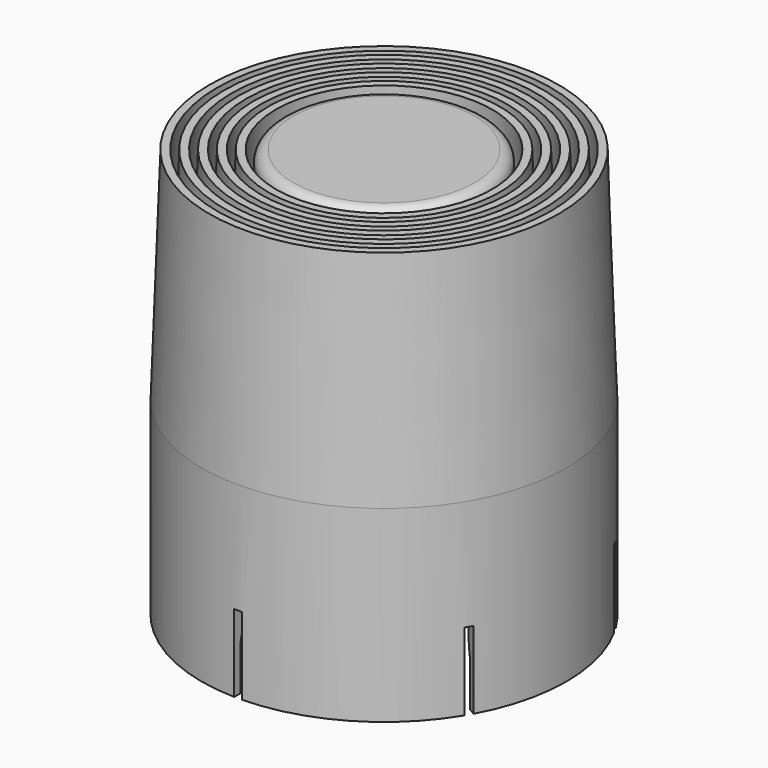
from build123d import *

# Parameters (mm, degrees)
F2_R     = 1
F4_DEPTH = 7


# Not quite as in the source:
# - a feature names something its author has since deleted; it is built from what else it names


with BuildPart() as f1:
    # F0 (on Front) → F1 (revolve)
    with BuildSketch(Plane.XZ):
        Polygon((-15.1, 10), (-15.8, 10), (-16.5, -10), (-15.8, -10), align=None)
        with BuildLine():
            Line((-15.8, -19), (-15.8, -23))
            ThreePointArc((-15.8, -23), (-15.5, -21), (-15.8, -19))
        make_face()
        with BuildLine():
            Line((-15.8, -10), (-16.5, -10))
            Line((-16.5, -10), (-16.5, -27))
            Line((-16.5, -27), (-15.8, -27))
            Line((-15.8, -27), (-15.8, -23))
            Line((-15.8, -23), (-15.8, -19))
            Line((-15.8, -19), (-15.8, -12.4))
            ThreePointArc((-15.8, -12.4), (-15.6828427125, -12.1171572875), (-15.4, -12))
            Line((-15.4, -12), (-14.6, -12))
            Line((-14.6, -12), (-15.8, -10))
        make_face()
    revolve(axis=Axis((0, 0, 4.5990636138), (0, 0, 1)))

    # F3 (on face) → F4 (cut)
    with BuildSketch(Plane(origin=(0, 0, -27), x_dir=(1, 0, 0), z_dir=(0, 0, -1))):
        Polygon((-0.35, -20), (0.35, -20), (0.35, -0.6062177826), (0, -0.4041451884), (-0.35, -0.6062177826), align=None)
        Polygon((0, -0.4041451884), (0.35, -0.6062177826), (0.35, -0.2020725942), align=None)
        Polygon((0.35, -0.2020725942), (0.35, -0.6062177826), (17.1455080757, -10.3031088913), (17.4955080757, -9.6968911087), (0.7, 0), align=None)
        Polygon((-17.1455080757, -10.3031088913), (-0.35, -0.6062177826), (-0.35, -0.2020725942), (-0.7, 0), (-17.4955080757, -9.6968911087), align=None)
        Polygon((-0.35, -0.2020725942), (-0.35, -0.6062177826), (0, -0.4041451884), align=None)
        Polygon((0.35, 0.2020725942), (0.35, -0.2020725942), (0.7, 0), align=None)
        Polygon((-0.7, 0), (-0.35, -0.2020725942), (-0.35, 0.2020725942), align=None)
        Polygon((0, 0.4041451884), (0.35, 0.2020725942), (0.35, 0.6062177826), align=None)
        Polygon((0.35, 0.6062177826), (0.35, 0.2020725942), (0.7, 0), (17.4955080757, 9.6968911087), (17.1455080757, 10.3031088913), align=None)
        Polygon((-0.7, 0), (-0.35, 0.2020725942), (-0.35, 0.6062177826), (-17.1455080757, 10.3031088913), (-17.4955080757, 9.6968911087), align=None)
        Polygon((-0.35, 0.6062177826), (-0.35, 0.2020725942), (0, 0.4041451884), align=None)
        Polygon((0, 0.4041451884), (0.35, 0.6062177826), (0.35, 20), (-0.35, 20), (-0.35, 0.6062177826), align=None)
    extrude(amount=-F4_DEPTH, mode=Mode.SUBTRACT)


with BuildPart() as f1b:
    # F0 (on Front) → F1, piece 2 (revolve)
    with BuildSketch(Plane.XZ):
        Polygon((-13.77, 10), (-14.47, 10), (-15.17, -10), (-14.47, -10), align=None)
    revolve(axis=Axis((0, 0, 4.5990636138), (0, 0, 1)))


with BuildPart() as f1c:
    # F0 (on Front) → F1, piece 3 (revolve)
    with BuildSketch(Plane.XZ):
        Polygon((-12.44, 10), (-13.14, 10), (-13.84, -10), (-13.14, -10), align=None)
    revolve(axis=Axis((0, 0, 4.5990636138), (0, 0, 1)))


with BuildPart() as f1d:
    # F0 (on Front) → F1, piece 4 (revolve)
    with BuildSketch(Plane.XZ):
        Polygon((-11.11, 10), (-11.81, 10), (-12.51, -10), (-11.81, -10), align=None)
    revolve(axis=Axis((0, 0, 4.5990636138), (0, 0, 1)))


with BuildPart() as f1e:
    # F0 (on Front) → F1, piece 5 (revolve)
    with BuildSketch(Plane.XZ):
        Polygon((-10.48, -10), (-9.78, 10), (-9.85, 10), (-10.48, 10), (-11.18, -10), align=None)
    revolve(axis=Axis((0, 0, 4.5990636138), (0, 0, 1)))


with BuildPart() as f1f:
    # F0 (on Front) → F1, piece 6 (revolve)
    with BuildSketch(Plane.XZ):
        Polygon((-9.1745, 9.3), (-9.85, -10), (-9.15, -10), (-8.4745, 9.3), align=None)
        Polygon((-9.15, 10), (-9.1745, 9.3), (-8.4745, 9.3), (-8.45, 10), align=None)
        Polygon((-8.45, 10), (-8.4745, 9.3), (0, 9.3), (0, 10), align=None)
    revolve(axis=Axis((0, 0, 4.5990636138), (0, 0, 1)))

    # F2
    f2_edges = [f1f.edges().sort_by_distance(p)[0] for p in [
        (9.15, 0, 10),
        (8.4745, 0, 9.3),
    ]]
    fillet(f2_edges, radius=F2_R)


solid = Compound([f1.part, f1b.part, f1c.part, f1d.part, f1e.part, f1f.part])
